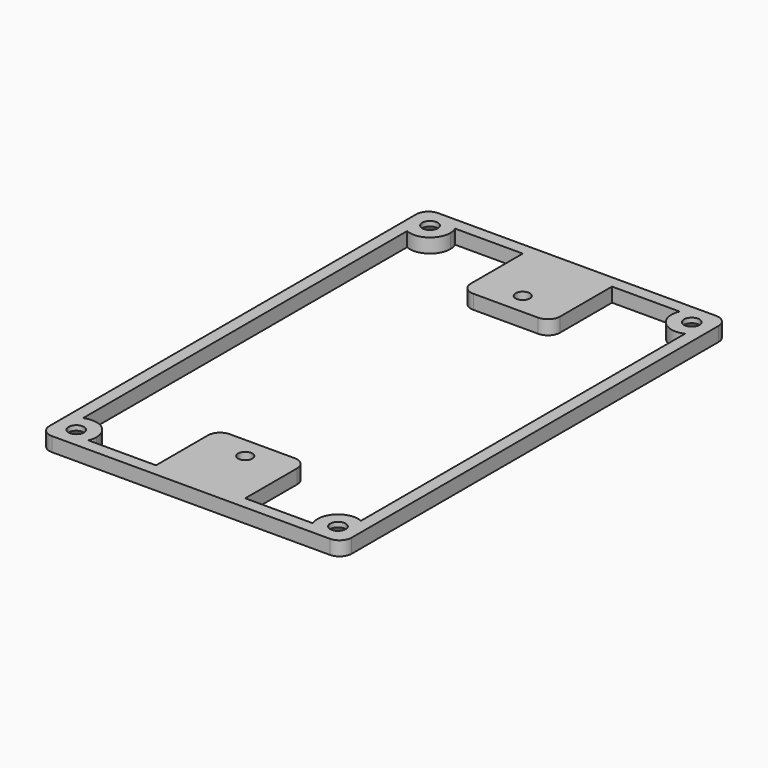
from build123d import *

# Parameters (mm, degrees)
F0_R           = 1.8985
F1_DEPTH       = 3.5
F2_R           = 3
F0_W           = 22
F0_H           = 19
F0_R_2         = 1.75
F3_DEPTH       = 3.5
F4_D           = 3.7973
F4_DEPTH       = 14.38125
F4_CSINK_D     = 7.7978
F4_CSINK_ANGLE = 82
F4_TIP         = 1.1408240143
F5_R           = 3


# Not quite as in the source:
# - a feature names something its author has since deleted; it is built from what else it names


with BuildPart() as f1:
    # F0 (on Top) → F1 (new body)
    with BuildSketch(Plane.XY):
        with BuildLine():
            Line((-32.25, 59.5), (-37.25, 59.5))
            Line((-37.25, 59.5), (-37.25, 54.5))
            ThreePointArc((-37.25, 54.5), (-35.7855339059, 58.0355339059), (-32.25, 59.5))
        make_face()
        with BuildLine():
            Line((37.25, 59.5), (32.25, 59.5))
            ThreePointArc((32.25, 59.5), (35.7855339059, 58.0355339059), (37.25, 54.5))
            Line((37.25, 54.5), (37.25, 59.5))
        make_face()
        with BuildLine():
            ThreePointArc((-32.25, -59.5), (-35.7855339059, -58.0355339059), (-37.25, -54.5))
            Line((-37.25, -54.5), (-37.25, -59.5))
            Line((-37.25, -59.5), (-32.25, -59.5))
        make_face()
        with BuildLine():
            Line((37.25, -59.5), (37.25, -54.5))
            ThreePointArc((37.25, -54.5), (35.7855339059, -58.0355339059), (32.25, -59.5))
            Line((32.25, -59.5), (37.25, -59.5))
        make_face()
        with BuildLine():
            Line((32.25, 59.5), (-32.25, 59.5))
            ThreePointArc((-32.25, 59.5), (-29.5113872125, 58.6833001327), (-27.667424305, 56.5))
            Line((-27.667424305, 56.5), (-11, 56.5))
            Line((-11, 56.5), (11, 56.5))
            Line((11, 56.5), (27.667424305, 56.5))
            ThreePointArc((27.667424305, 56.5), (29.5113872125, 58.6833001327), (32.25, 59.5))
        make_face()
        with BuildLine():
            ThreePointArc((-27.667424305, -56.5), (-29.5113872125, -58.6833001327), (-32.25, -59.5))
            Line((-32.25, -59.5), (32.25, -59.5))
            ThreePointArc((32.25, -59.5), (29.5113872125, -58.6833001327), (27.667424305, -56.5))
            Line((27.667424305, -56.5), (11, -56.5))
            Line((11, -56.5), (-11, -56.5))
            Line((-11, -56.5), (-27.667424305, -56.5))
        make_face()
        with BuildLine():
            ThreePointArc((-34.25, 49.917424305), (-36.4333001327, 51.7613872125), (-37.25, 54.5))
            Line((-37.25, 54.5), (-37.25, -54.5))
            ThreePointArc((-37.25, -54.5), (-36.4333001327, -51.7613872125), (-34.25, -49.917424305))
            Line((-34.25, -49.917424305), (-34.25, 49.917424305))
        make_face()
        with BuildLine():
            Line((37.25, -54.5), (37.25, 54.5))
            ThreePointArc((37.25, 54.5), (36.4333001327, 51.7613872125), (34.25, 49.917424305))
            Line((34.25, 49.917424305), (34.25, -49.917424305))
            ThreePointArc((34.25, -49.917424305), (36.4333001327, -51.7613872125), (37.25, -54.5))
        make_face()
        with BuildLine():
            ThreePointArc((-27.667424305, 56.5), (-29.5113872125, 58.6833001327), (-32.25, 59.5))
            ThreePointArc((-32.25, 59.5), (-35.7855339059, 58.0355339059), (-37.25, 54.5))
            ThreePointArc((-37.25, 54.5), (-36.4333001327, 51.7613872125), (-34.25, 49.917424305))
            Line((-34.25, 49.917424305), (-34.25, 56.5))
            Line((-34.25, 56.5), (-27.667424305, 56.5))
        make_face()
        with BuildLine():
            ThreePointArc((32.25, -59.5), (35.7855339059, -58.0355339059), (37.25, -54.5))
            ThreePointArc((37.25, -54.5), (36.4333001327, -51.7613872125), (34.25, -49.917424305))
            Line((34.25, -49.917424305), (34.25, -56.5))
            Line((34.25, -56.5), (27.667424305, -56.5))
            ThreePointArc((27.667424305, -56.5), (29.5113872125, -58.6833001327), (32.25, -59.5))
        make_face()
        with BuildLine():
            ThreePointArc((-27.25, 54.5), (-27.3554684353, 55.5215482184), (-27.667424305, 56.5))
            Line((-27.667424305, 56.5), (-34.25, 56.5))
            Line((-34.25, 56.5), (-34.25, 49.917424305))
            ThreePointArc((-34.25, 49.917424305), (-29.5113872125, 50.3166998673), (-27.25, 54.5))
        make_face()
        with Locations((-32.25, 54.5)):
            Circle(F0_R, mode=Mode.SUBTRACT)
        with BuildLine():
            ThreePointArc((-27.25, -54.5), (-29.5113872125, -50.3166998673), (-34.25, -49.917424305))
            Line((-34.25, -49.917424305), (-34.25, -56.5))
            Line((-34.25, -56.5), (-27.667424305, -56.5))
            ThreePointArc((-27.667424305, -56.5), (-27.3554684353, -55.5215482184), (-27.25, -54.5))
        make_face()
        with Locations((-32.25, -54.5)):
            Circle(F0_R, mode=Mode.SUBTRACT)
        with BuildLine():
            ThreePointArc((-34.25, -49.917424305), (-36.4333001327, -51.7613872125), (-37.25, -54.5))
            ThreePointArc((-37.25, -54.5), (-35.7855339059, -58.0355339059), (-32.25, -59.5))
            ThreePointArc((-32.25, -59.5), (-29.5113872125, -58.6833001327), (-27.667424305, -56.5))
            Line((-27.667424305, -56.5), (-34.25, -56.5))
            Line((-34.25, -56.5), (-34.25, -49.917424305))
        make_face()
        with BuildLine():
            Line((34.25, -56.5), (34.25, -49.917424305))
            ThreePointArc((34.25, -49.917424305), (28.7144660941, -50.9644660941), (27.667424305, -56.5))
            Line((27.667424305, -56.5), (34.25, -56.5))
        make_face()
        with Locations((32.25, -54.5)):
            Circle(F0_R, mode=Mode.SUBTRACT)
        with BuildLine():
            Line((34.25, 56.5), (27.667424305, 56.5))
            ThreePointArc((27.667424305, 56.5), (28.7144660941, 50.9644660941), (34.25, 49.917424305))
            Line((34.25, 49.917424305), (34.25, 56.5))
        make_face()
        with Locations((32.25, 54.5)):
            Circle(F0_R, mode=Mode.SUBTRACT)
        with BuildLine():
            ThreePointArc((37.25, 54.5), (35.7855339059, 58.0355339059), (32.25, 59.5))
            ThreePointArc((32.25, 59.5), (29.5113872125, 58.6833001327), (27.667424305, 56.5))
            Line((27.667424305, 56.5), (34.25, 56.5))
            Line((34.25, 56.5), (34.25, 49.917424305))
            ThreePointArc((34.25, 49.917424305), (36.4333001327, 51.7613872125), (37.25, 54.5))
        make_face()
        with Locations((-32.25, 54.5)):
            Circle(F0_R)
        with Locations((32.25, 54.5)):
            Circle(F0_R)
        with Locations((-32.25, -54.5)):
            Circle(F0_R)
        with Locations((32.25, -54.5)):
            Circle(F0_R)
    extrude(amount=F1_DEPTH)

    # F2
    f2_edges = [f1.edges().sort_by_distance(p)[0] for p in [
        (-37.25, 59.5, 1.75),
        (37.25, 59.5, 1.75),
        (37.25, -59.5, 1.75),
        (-37.25, -59.5, 1.75),
    ]]
    fillet(f2_edges, radius=F2_R)

    # F0 (on Top) → F3 (join)
    with BuildSketch(Plane.XY):
        with Locations((0, 47)):
            Rectangle(F0_W, F0_H)
        with Locations((0, 42.75)):
            Circle(F0_R_2, mode=Mode.SUBTRACT)
        with Locations((0, -47)):
            Rectangle(F0_W, F0_H)
        with Locations((0, -42.75)):
            Circle(F0_R_2, mode=Mode.SUBTRACT)
    extrude(amount=F3_DEPTH)

    # F4
    with Locations(Plane(origin=(0, 0, 0), x_dir=(1, 0, 0), z_dir=(0, 0, -1))):
        with Locations((-32.25, -54.5), (32.25, -54.5), (32.25, 54.5), (-32.25, 54.5)):
            CounterSinkHole(F4_D / 2, F4_CSINK_D / 2, depth=F4_DEPTH, counter_sink_angle=F4_CSINK_ANGLE)
            with Locations((0, 0, -(F4_DEPTH + F4_TIP / 2))):  # 118° drill point
                Cone(0, F4_D / 2, F4_TIP, mode=Mode.SUBTRACT)

    # F5
    f5_edges = [f1.edges().sort_by_distance(p)[0] for p in [
        (-11, 37.5, 1.75),
        (11, 37.5, 1.75),
        (11, -37.5, 1.75),
        (-11, -37.5, 1.75),
    ]]
    fillet(f5_edges, radius=F5_R)


solid = f1.part
